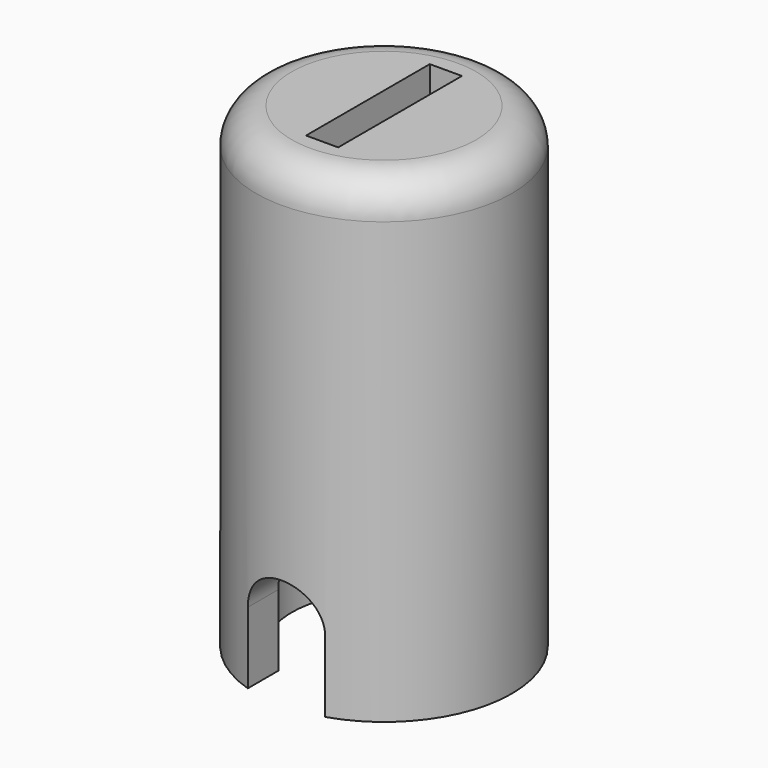
from build123d import *

# Parameters (mm, degrees)
F0_R     = 10.75
F0_R_2   = 7.75
F1_DEPTH = 40
F3_DEPTH = 15
F4_DEPTH = 25
F7_R     = 3
F6_W     = 2.7
F6_H     = 13
F8_DEPTH = 25


# Not quite as in the source:
# - a fillet or chamfer that OpenCascade refuses, or shapes differently, is made with other operations: its cross-section is extruded or revolved along the edge and cut away or added


with BuildPart() as f1:
    # F0 (on Top) → F1 (new body)
    with BuildSketch(Plane.XY):
        Circle(F0_R)
        Circle(F0_R_2, mode=Mode.SUBTRACT)
        Circle(F0_R_2)
    extrude(amount=F1_DEPTH)

    # F2 (on Front) → F3 (cut)
    with BuildSketch(Plane.XZ):
        with BuildLine():
            Line((-3.25, 6), (-3.25, 0))
            Line((-3.25, 0), (3.25, 0))
            Line((3.25, 0), (3.25, 6))
            ThreePointArc((3.25, 6), (0, 9.25), (-3.25, 6))
        make_face()
    extrude(amount=F3_DEPTH, mode=Mode.SUBTRACT)

    # F0 (on Top) → F4 (cut)
    with BuildSketch(Plane.XY):
        Circle(F0_R_2)
    extrude(amount=F4_DEPTH, mode=Mode.SUBTRACT)

    # F7
    f7_edges = [f1.edges().sort_by_distance(p)[0] for p in [
        (-10.75, 0, 40),
    ]]
    fillet(f7_edges, radius=F7_R)

    # F6 (on offset) → F8 (cut)
    with BuildSketch(Plane.XY.offset(40)):
        Rectangle(F6_W, F6_H)
    extrude(amount=-F8_DEPTH, mode=Mode.SUBTRACT)

    # F9: fillet of radius 4 on 1 edges, made by hand


with BuildPart() as f9_tool2:
    # F9_s3 → F9_t4 (revolve)
    with BuildSketch(Plane.XZ):
        with BuildLine():
            ThreePointArc((7.75, 21), (6.5784271247, 23.8284271247), (3.75, 25))
            Line((3.75, 25), (7.75, 25))
            Line((7.75, 25), (7.75, 21))
        make_face()
    revolve(axis=Axis((0, 0, 25), (0, 0, 1)))

    split(bisect_by=Plane.YZ.offset(1.35), keep=Keep.TOP)


with BuildPart() as f1_1:
    add(f1.part)

    # F9_t1: union F9_tool2
    add(f9_tool2.part)


with BuildPart() as f9_tool7:
    # F9_s8 → F9_t9 (revolve)
    with BuildSketch(Plane.XZ):
        with BuildLine():
            ThreePointArc((7.75, 21), (6.5784271247, 23.8284271247), (3.75, 25))
            Line((3.75, 25), (7.75, 25))
            Line((7.75, 25), (7.75, 21))
        make_face()
    revolve(axis=Axis((0, 0, 25), (0, 0, 1)))

    split(bisect_by=Plane.YZ.offset(-1.35), keep=Keep.BOTTOM)


with BuildPart() as f1_2:
    add(f1_1.part)

    # F9_t6: union F9_tool7
    add(f9_tool7.part)


with BuildPart() as f9_tool12:
    # F9_s13 → F9_t14 (revolve)
    with BuildSketch(Plane.XZ):
        with BuildLine():
            ThreePointArc((7.75, 21), (6.5784271247, 23.8284271247), (3.75, 25))
            Line((3.75, 25), (7.75, 25))
            Line((7.75, 25), (7.75, 21))
        make_face()
    revolve(axis=Axis((0, 0, 25), (0, 0, 1)))

    split(bisect_by=Plane.XZ.offset(-6.5), keep=Keep.BOTTOM)


with BuildPart() as f1_3:
    add(f1_2.part)

    # F9_t11: union F9_tool12
    add(f9_tool12.part)


with BuildPart() as f9_tool17:
    # F9_s18 → F9_t19 (revolve)
    with BuildSketch(Plane.XZ):
        with BuildLine():
            ThreePointArc((7.75, 21), (6.5784271247, 23.8284271247), (3.75, 25))
            Line((3.75, 25), (7.75, 25))
            Line((7.75, 25), (7.75, 21))
        make_face()
    revolve(axis=Axis((0, 0, 25), (0, 0, 1)))

    split(bisect_by=Plane.XZ.offset(6.5), keep=Keep.TOP)


with BuildPart() as f1_4:
    add(f1_3.part)

    # F9_t16: union F9_tool17
    add(f9_tool17.part)


solid = f1_4.part
